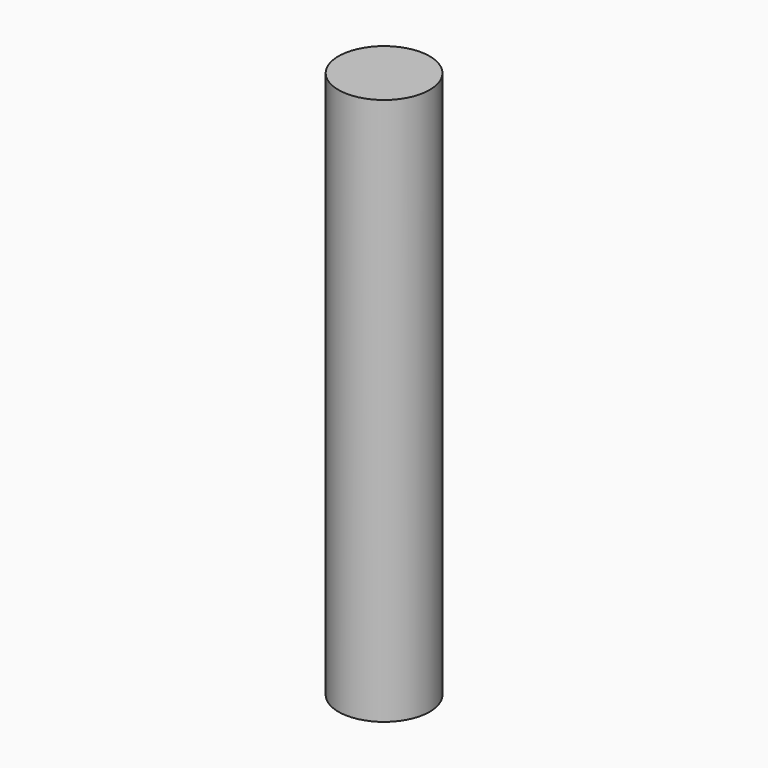
from build123d import *

# Parameters (mm, degrees)
F1_R     = 3.175
F2_DEPTH = 38.1


# Not quite as in the source:
# - a variable given as a bare number and used for a length is read in inches; the dataset says mm whatever the document's units were


with BuildPart() as f2:
    # F1 (on Top) → F2 (new body)
    with BuildSketch(Plane.XY):
        Circle(F1_R)
    extrude(amount=F2_DEPTH)


solid = f2.part
